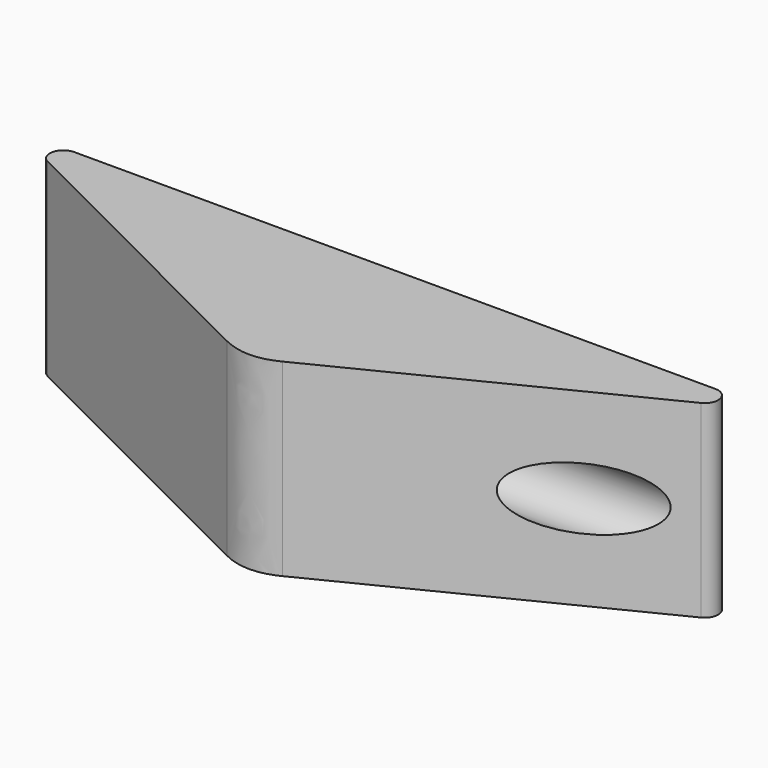
from build123d import *

# Parameters (mm, degrees)
F1_DEPTH    = 70
F2_R        = 5
F3_T1_DEPTH = 127.5
F5_D        = 23
F5_DEPTH    = 123.8206602125


# Not quite as in the source:
# - a fillet or chamfer that OpenCascade refuses, or shapes differently, is made with other operations: its cross-section is extruded or revolved along the edge and cut away or added


with BuildPart() as f1:
    # F0 (on Top) → F1 (new body)
    with BuildSketch(Plane.XY):
        Polygon((140, 70), (-140, 70), (0, 0), align=None)
    extrude(amount=F1_DEPTH)

    # F2
    f2_edges = [f1.edges().sort_by_distance(p)[0] for p in [
        (140, 70, 35),
        (-140, 70, 35),
    ]]
    fillet(f2_edges, radius=F2_R)

    # F3: fillet of radius 23 on 1 edges, made by hand

    # F3_s2 → F3_t1 (cut)
    with BuildSketch(Plane.XY.offset(-28.75)):
        with BuildLine():
            add(Edge.make_bspline(
                [(10.2859126965, 5.1429563482), (0, 0), (-10.2859126965, 5.1429563482)],
                knots=[0, 0, 0, 1, 1, 1], degree=2, weights=[1, 1, 1]))
            Line((-10.2859126965, 5.1429563482), (0, 0))
            Line((0, 0), (10.2859126965, 5.1429563482))
        make_face()
    extrude(amount=F3_T1_DEPTH, mode=Mode.SUBTRACT)

    # F5 (through all, one way)
    with BuildSketch(Plane(origin=(0, 0, 0), x_dir=(0, 1, 0), z_dir=(-1, 0, 0))):
        with Locations((45, -35)):
            Circle(F5_D / 2)
    extrude(amount=-F5_DEPTH, mode=Mode.SUBTRACT)


solid = f1.part
